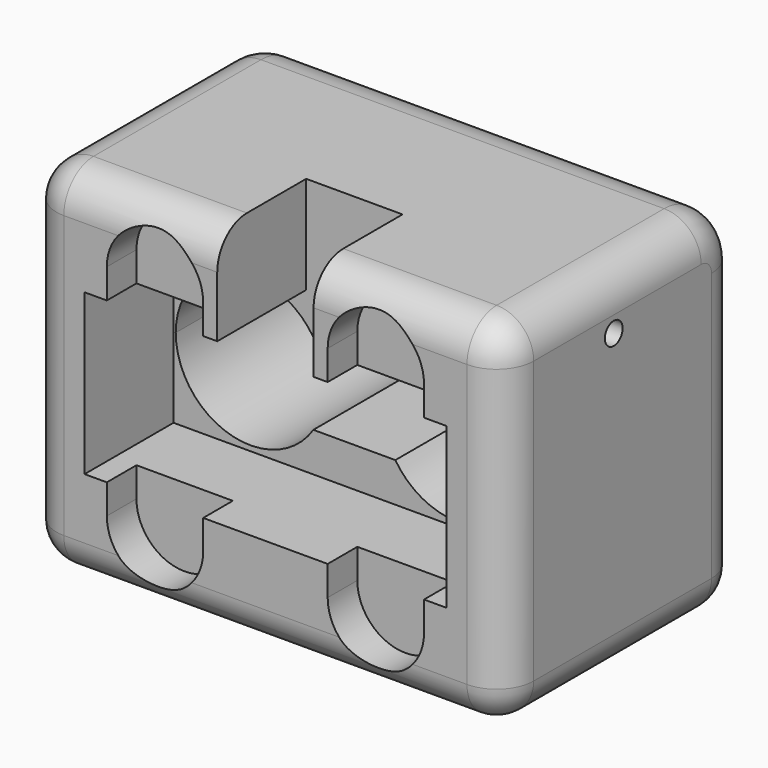
from build123d import *

# Parameters (mm, degrees)
F1_DEPTH      = 5
F3_DEPTH      = 10
F5_DEPTH      = 25
F6_R          = 1.5
F7_DEPTH      = 69.4
F8_R          = 6.7597979746
F9_R          = 5
F10_R         = 5
F11_T1_DEPTH  = 45.7
F11_T3_DEPTH  = 45.7
F12_T1_DEPTH  = 54.4
F12_T3_DEPTH  = 30
F12_T5_DEPTH  = 38
F12_S9_W      = 5
F12_S9_H      = 5
F12_T10_DEPTH = 5
F12_S15_W     = 5
F12_S15_H     = 5
F12_T16_DEPTH = 5
F12_S21_W     = 5
F12_S21_H     = 5
F12_T22_DEPTH = 5
F12_S27_W     = 5
F12_S27_H     = 5
F12_T28_DEPTH = 5
F12_T32_ANGLE = 90
F12_T34_ANGLE = 90


# Not quite as in the source:
# - a fillet or chamfer that OpenCascade refuses, or shapes differently, is made with other operations: its cross-section is extruded or revolved along the edge and cut away or added


with BuildPart() as f1:
    # F0 (on Front) → F1 (new body)
    with BuildSketch(Plane.XZ):
        with BuildLine():
            Line((32.2, -24), (32.2, 24))
            Line((32.2, 24), (6.5, 24))
            Line((6.5, 24), (6.5, 10.8))
            Line((6.5, 10.8), (8.4, 10.8))
            Line((8.4, 10.8), (8.4, 14.8))
            ThreePointArc((8.4, 14.8), (14.9, 21.3), (21.4, 14.8))
            Line((21.4, 14.8), (21.4, 10.8))
            Line((21.4, 10.8), (24.4, 10.8))
            Line((24.4, 10.8), (24.4, -10.8))
            Line((24.4, -10.8), (21.4, -10.8))
            Line((21.4, -10.8), (21.4, -14.8))
            ThreePointArc((21.4, -14.8), (14.9, -21.3), (8.4, -14.8))
            Line((8.4, -14.8), (8.4, -10.8))
            Line((8.4, -10.8), (-8.4, -10.8))
            Line((-8.4, -10.8), (-8.4, -14.8))
            ThreePointArc((-8.4, -14.8), (-14.9, -21.3), (-21.4, -14.8))
            Line((-21.4, -14.8), (-21.4, -10.8))
            Line((-21.4, -10.8), (-24.4, -10.8))
            Line((-24.4, -10.8), (-24.4, 10.8))
            Line((-24.4, 10.8), (-21.4, 10.8))
            Line((-21.4, 10.8), (-21.4, 14.8))
            ThreePointArc((-21.4, 14.8), (-14.9, 21.3), (-8.4, 14.8))
            Line((-8.4, 14.8), (-8.4, 10.8))
            Line((-8.4, 10.8), (-6.5, 10.8))
            Line((-6.5, 10.8), (-6.5, 24))
            Line((-6.5, 24), (-32.2, 24))
            Line((-32.2, 24), (-32.2, -24))
            Line((-32.2, -24), (32.2, -24))
        make_face()
    extrude(amount=F1_DEPTH)

    # F2 (on face) → F3 (join)
    with BuildSketch(Plane(origin=(0, 0, 0), x_dir=(-1, 0, 0), z_dir=(0, 1, 0))):
        with BuildLine():
            Line((24.4, 10.8), (24.4, -10.8))
            Line((24.4, -10.8), (21.4, -10.8))
            Line((21.4, -10.8), (21.4, -14.8))
            ThreePointArc((21.4, -14.8), (14.9, -21.3), (8.4, -14.8))
            Line((8.4, -14.8), (8.4, -10.8))
            Line((8.4, -10.8), (-8.4, -10.8))
            Line((-8.4, -10.8), (-8.4, -14.8))
            ThreePointArc((-8.4, -14.8), (-14.9, -21.3), (-21.4, -14.8))
            Line((-21.4, -14.8), (-21.4, -10.8))
            Line((-21.4, -10.8), (-24.4, -10.8))
            Line((-24.4, -10.8), (-24.4, 10.8))
            Line((-24.4, 10.8), (-21.4, 10.8))
            Line((-21.4, 10.8), (-21.4, 14.8))
            ThreePointArc((-21.4, 14.8), (-14.9, 21.3), (-8.4, 14.8))
            Line((-8.4, 14.8), (-8.4, 10.8))
            Line((-8.4, 10.8), (-6.5, 10.8))
            Line((-6.5, 10.8), (-6.5, 24))
            Line((-6.5, 24), (-32.2, 24))
            Line((-32.2, 24), (-32.2, -24))
            Line((-32.2, -24), (32.2, -24))
            Line((32.2, -24), (32.2, 24))
            Line((32.2, 24), (6.5, 24))
            Line((6.5, 24), (6.5, 10.8))
            Line((6.5, 10.8), (8.4, 10.8))
            Line((8.4, 10.8), (8.4, 14.8))
            ThreePointArc((8.4, 14.8), (14.9, 21.3), (21.4, 14.8))
            Line((21.4, 14.8), (21.4, 10.8))
            Line((21.4, 10.8), (24.4, 10.8))
        make_face()
        with BuildLine():
            Line((21.4, -14.8), (21.4, -10.8))
            Line((21.4, -10.8), (8.4, -10.8))
            Line((8.4, -10.8), (8.4, -14.8))
            ThreePointArc((8.4, -14.8), (14.9, -21.3), (21.4, -14.8))
        make_face()
        with BuildLine():
            Line((-8.4, -14.8), (-8.4, -10.8))
            Line((-8.4, -10.8), (-21.4, -10.8))
            Line((-21.4, -10.8), (-21.4, -14.8))
            ThreePointArc((-21.4, -14.8), (-14.9, -21.3), (-8.4, -14.8))
        make_face()
        with BuildLine():
            Line((8.4, 10.8), (21.4, 10.8))
            Line((21.4, 10.8), (21.4, 14.8))
            ThreePointArc((21.4, 14.8), (14.9, 21.3), (8.4, 14.8))
            Line((8.4, 14.8), (8.4, 10.8))
        make_face()
        with BuildLine():
            Line((-21.4, 10.8), (-8.4, 10.8))
            Line((-8.4, 10.8), (-8.4, 14.8))
            ThreePointArc((-8.4, 14.8), (-14.9, 21.3), (-21.4, 14.8))
            Line((-21.4, 14.8), (-21.4, 10.8))
        make_face()
    extrude(amount=F3_DEPTH)

    # F4 (on face) → F5 (join)
    with BuildSketch(Plane(origin=(0, 10, 0), x_dir=(-1, 0, 0), z_dir=(0, 1, 0))):
        Polygon((32.2, -24), (32.2, 24), (6.5, 24), (6.5, 10.8), (24.4, 10.8), (24.4, -10.8), (-24.4, -10.8), (-24.4, 10.8), (-6.5, 10.8), (-6.5, 24), (-32.2, 24), (-32.2, -24), align=None)
        Polygon((6.5, 10.8), (6.5, 24), (-6.5, 24), (-6.5, 10.8), (-24.4, 10.8), (-24.4, -10.8), (24.4, -10.8), (24.4, 10.8), align=None)
        with BuildLine():
            ThreePointArc((5.5288725662, 5.5), (16.8680666762, 9.6842239514), (24.1, 0))
            ThreePointArc((24.1, 0), (16.8680666762, -9.6842239514), (5.5288725662, -5.5))
            Line((5.5288725662, -5.5), (0, -5.5))
            Line((0, -5.5), (-5.5288725662, -5.5))
            ThreePointArc((-5.5288725662, -5.5), (-24.1, 0), (-5.5288725662, 5.5))
            Line((-5.5288725662, 5.5), (0, 5.5))
            Line((0, 5.5), (5.5288725662, 5.5))
        make_face(mode=Mode.SUBTRACT)
    extrude(amount=F5_DEPTH)

    # F6 (on face) → F7 (cut)
    with BuildSketch(Plane(origin=(-32.2, 0, 0), x_dir=(0, -1, 0), z_dir=(-1, 0, 0))):
        with Locations((-13.5, 16.806252715)):
            Circle(F6_R)
    extrude(amount=-F7_DEPTH, mode=Mode.SUBTRACT)

    # F8
    f8_edges = [f1.edges().sort_by_distance(p)[0] for p in [
        (0, 35, 24),
    ]]
    fillet(f8_edges, radius=F8_R)

    # F9
    f9_edges = [f1.edges().sort_by_distance(p)[0] for p in [
        (32.2, 33.020101, 22.020101),
        (32.2, 35, -3.379899),
    ]]
    fillet(f9_edges, radius=F9_R)

    # F10
    f10_edges = [f1.edges().sort_by_distance(p)[0] for p in [
        (-32.2, 35, -3.379899),
    ]]
    fillet(f10_edges, radius=F10_R)

    # F11: fillet of radius 5 on 2 edges, made by hand

    # F11_s2 → F11_t1 (cut)
    with BuildSketch(Plane.YZ.offset(-39.7)):
        with BuildLine():
            ThreePointArc((-5, 19), (-3.5355339059, 22.5355339059), (0, 24))
            Line((0, 24), (-5, 24))
            Line((-5, 24), (-5, 19))
        make_face()
    extrude(amount=F11_T1_DEPTH, mode=Mode.SUBTRACT)

    # F11_s4 → F11_t3 (cut)
    with BuildSketch(Plane.YZ.offset(-6)):
        with BuildLine():
            ThreePointArc((-5, 19), (-3.5355339059, 22.5355339059), (0, 24))
            Line((0, 24), (-5, 24))
            Line((-5, 24), (-5, 19))
        make_face()
    extrude(amount=F11_T3_DEPTH, mode=Mode.SUBTRACT)

    # F12: fillet of radius 5 on 8 edges, made by hand

    # F12_s2 → F12_t1 (cut)
    with BuildSketch(Plane.YZ.offset(-27.2)):
        with BuildLine():
            ThreePointArc((30, -24), (33.5355339059, -22.5355339059), (35, -19))
            Line((35, -19), (35, -24))
            Line((35, -24), (30, -24))
        make_face()
        with BuildLine():
            ThreePointArc((0, -24), (-3.5355339059, -22.5355339059), (-5, -19))
            Line((-5, -19), (-5, -24))
            Line((-5, -24), (0, -24))
        make_face()
    extrude(amount=F12_T1_DEPTH, mode=Mode.SUBTRACT)

    # F12_s4 → F12_t3 (cut)
    with BuildSketch(Plane.XZ.offset(-30)):
        with BuildLine():
            ThreePointArc((-27.2, -24), (-30.7355339059, -22.5355339059), (-32.2, -19))
            Line((-32.2, -19), (-32.2, -24))
            Line((-32.2, -24), (-27.2, -24))
        make_face()
        with BuildLine():
            ThreePointArc((27.2, -24), (30.7355339059, -22.5355339059), (32.2, -19))
            Line((32.2, -19), (32.2, -24))
            Line((32.2, -24), (27.2, -24))
        make_face()
    extrude(amount=F12_T3_DEPTH, mode=Mode.SUBTRACT)

    # F12_s6 → F12_t5 (cut)
    with BuildSketch(Plane.XY.offset(-19)):
        with BuildLine():
            ThreePointArc((-32.2, 0), (-30.7355339059, -3.5355339059), (-27.2, -5))
            Line((-27.2, -5), (-32.2, -5))
            Line((-32.2, -5), (-32.2, 0))
        make_face()
        with BuildLine():
            ThreePointArc((32.2, 0), (30.7355339059, -3.5355339059), (27.2, -5))
            Line((27.2, -5), (32.2, -5))
            Line((32.2, -5), (32.2, 0))
        make_face()
    extrude(amount=F12_T5_DEPTH, mode=Mode.SUBTRACT)


with BuildPart() as f12_tool8:
    # F12_s9 → F12_t10 (new body)
    with BuildSketch(Plane.YZ.offset(27.2)):
        with Locations((-2.5, 21.5)):
            Rectangle(F12_S9_W, F12_S9_H)
    extrude(amount=F12_T10_DEPTH)

    # F12_s11 → F12_t12 (revolve, cut)
    with BuildSketch(Plane(origin=(27.2, 0, 19), x_dir=(0, 0.7071067812, -0.7071067812), z_dir=(0, -0.7071067812, -0.7071067812))):
        with BuildLine():
            ThreePointArc((0, -5), (5, 0), (0, 5))
            Line((0, 5), (0, -5))
        make_face()
    revolve(axis=Axis((27.2, 0, 19), (1, 0, 0)), mode=Mode.SUBTRACT)


with BuildPart() as f1_1:
    add(f1.part)

    # F12_t7: cut F12_tool8
    add(f12_tool8.part, mode=Mode.SUBTRACT)


with BuildPart() as f12_tool14:
    # F12_s15 → F12_t16 (new body)
    with BuildSketch(Plane.YZ.offset(-27.2)):
        with Locations((-2.5, 21.5)):
            Rectangle(F12_S15_W, F12_S15_H)
    extrude(amount=-F12_T16_DEPTH)

    # F12_s17 → F12_t18 (revolve, cut)
    with BuildSketch(Plane(origin=(-27.2, 0, 19), x_dir=(0, 0.7071067812, -0.7071067812), z_dir=(0, 0.7071067812, 0.7071067812))):
        with BuildLine():
            ThreePointArc((0, -5), (5, 0), (0, 5))
            Line((0, 5), (0, -5))
        make_face()
    revolve(axis=Axis((-27.2, 0, 19), (-1, 0, 0)), mode=Mode.SUBTRACT)


with BuildPart() as f1_2:
    add(f1_1.part)

    # F12_t13: cut F12_tool14
    add(f12_tool14.part, mode=Mode.SUBTRACT)


with BuildPart() as f12_tool20:
    # F12_s21 → F12_t22 (new body)
    with BuildSketch(Plane.XY.offset(-19)):
        with Locations((-29.7, -2.5)):
            Rectangle(F12_S21_W, F12_S21_H)
    extrude(amount=-F12_T22_DEPTH)

    # F12_s23 → F12_t24 (revolve, cut)
    with BuildSketch(Plane(origin=(-27.2, 0, -19), x_dir=(0.7071067812, 0.7071067812, 0), z_dir=(-0.7071067812, 0.7071067812, 0))):
        with BuildLine():
            ThreePointArc((0, -5), (5, 0), (0, 5))
            Line((0, 5), (0, -5))
        make_face()
    revolve(axis=Axis((-27.2, 0, -19), (0, 0, -1)), mode=Mode.SUBTRACT)


with BuildPart() as f1_3:
    add(f1_2.part)

    # F12_t19: cut F12_tool20
    add(f12_tool20.part, mode=Mode.SUBTRACT)


with BuildPart() as f12_tool26:
    # F12_s27 → F12_t28 (new body)
    with BuildSketch(Plane.XY.offset(-19)):
        with Locations((29.7, -2.5)):
            Rectangle(F12_S27_W, F12_S27_H)
    extrude(amount=-F12_T28_DEPTH)

    # F12_s29 → F12_t30 (revolve, cut)
    with BuildSketch(Plane(origin=(27.2, 0, -19), x_dir=(-0.7071067812, 0.7071067812, 0), z_dir=(-0.7071067812, -0.7071067812, 0))):
        with BuildLine():
            ThreePointArc((0, -5), (5, 0), (0, 5))
            Line((0, 5), (0, -5))
        make_face()
    revolve(axis=Axis((27.2, 0, -19), (0, 0, -1)), mode=Mode.SUBTRACT)


with BuildPart() as f1_4:
    add(f1_3.part)

    # F12_t25: cut F12_tool26
    add(f12_tool26.part, mode=Mode.SUBTRACT)

    # F12_s31 → F12_t32 (revolve, cut)
    with BuildSketch(Plane.YZ.offset(-27.2)):
        with BuildLine():
            ThreePointArc((30, -24), (33.5355339059, -22.5355339059), (35, -19))
            Line((35, -19), (35, -24))
            Line((35, -24), (30, -24))
        make_face()
    revolve(axis=Axis((-27.2, 30, -24), (0, 0, 1)), revolution_arc=F12_T32_ANGLE, mode=Mode.SUBTRACT)

    # F12_s33 → F12_t34 (revolve, cut)
    with BuildSketch(Plane.XZ.offset(-30)):
        with BuildLine():
            ThreePointArc((27.2, -24), (30.7355339059, -22.5355339059), (32.2, -19))
            Line((32.2, -19), (32.2, -24))
            Line((32.2, -24), (27.2, -24))
        make_face()
    revolve(axis=Axis((27.2, 30, -24), (0, 0, 1)), revolution_arc=F12_T34_ANGLE, mode=Mode.SUBTRACT)


solid = f1_4.part
